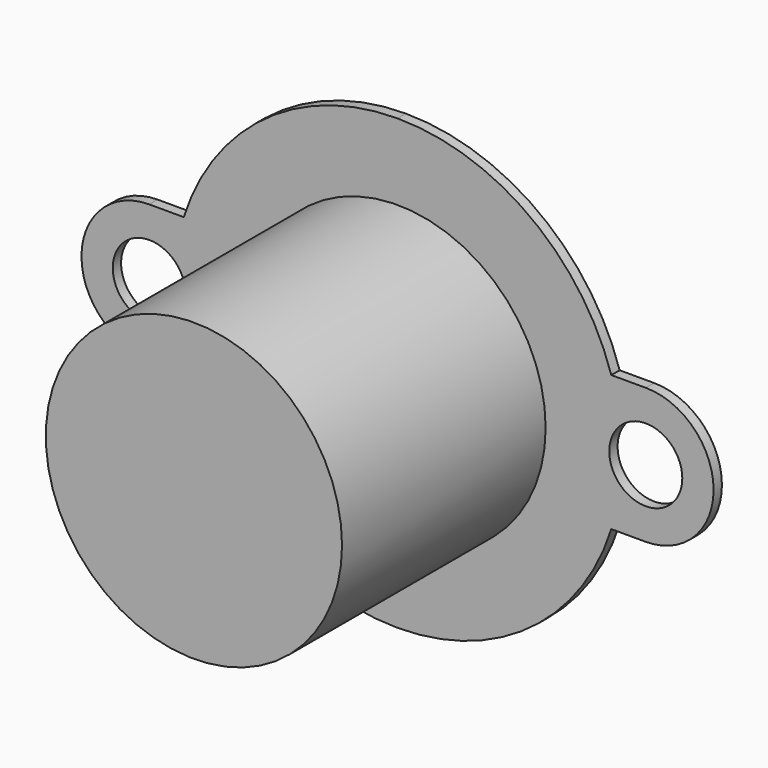
from build123d import *

# Parameters (mm, degrees)
F0_R     = 7.1
F1_DEPTH = 12.7
F2_R     = 1.75
F3_DEPTH = 0.5


# Not quite as in the source:
# - ends of sketch curves that miss each other by under 0.0002 mm in the source are joined


with BuildPart() as f1:
    # F0 (on Front) → F1 (new body)
    with BuildSketch(Plane.XZ):
        Circle(F0_R)
    extrude(amount=F1_DEPTH)

    # F2 (on Front) → F3 (join)
    with BuildSketch(Plane.XZ):
        with BuildLine():
            Line((10.246950766, -3.25), (11.9, -3.25))
            ThreePointArc((11.9, -3.25), (15.15, 0), (11.9, 3.25))
            Line((11.9, 3.25), (10.2469522811, 3.25))
            ThreePointArc((10.2469522811, 3.25), (6.3492135874, 8.6746768166), (0, 10.7500014442))
            ThreePointArc((0, 10.7500014442), (-6.3492135874, 8.6746768166), (-10.2469522811, 3.25))
            Line((-10.2469522811, 3.25), (-11.9, 3.249995223))
            Line((-11.9, 3.249995223), (-11.9055723148, 3.249995223))
            ThreePointArc((-11.9055723148, 3.249995223), (-15.1499988057, -0.0027861584), (-11.9, -3.25))
            Line((-11.9, -3.25), (-10.246950766, -3.25))
            ThreePointArc((-10.246950766, -3.25), (-6.3492125496, -8.6746757864), (0, -10.75))
            ThreePointArc((0, -10.75), (6.3492125496, -8.6746757864), (10.246950766, -3.25))
        make_face()
        with Locations((-11.9, 0)):
            Circle(F2_R, mode=Mode.SUBTRACT)
        with Locations((11.9, 0)):
            Circle(F2_R, mode=Mode.SUBTRACT)
    extrude(amount=F3_DEPTH)


solid = f1.part
